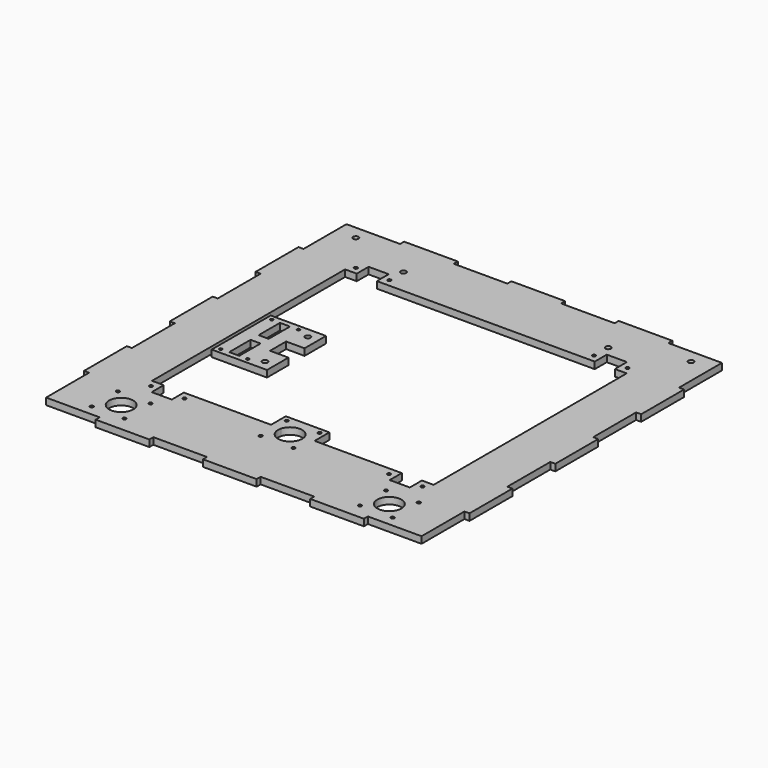
from build123d import *

# Parameters (mm, degrees)
F0_R     = 1.5875
F0_R_2   = 11.43
F0_R_3   = 3.175
F0_W     = 4.7625
F0_H     = 50.8
F0_W_2   = 50.8
F0_H_2   = 4.7625
F0_W_3   = 44.45
F0_H_3   = 41.1268851364
F1_DEPTH = 6.35
F0_R_4   = 1.8415
F0_W_4   = 9.525
F0_H_4   = 25.273
F0_W_5   = 17.4625
F0_H_5   = 25.4
F2_D     = 2.7051
F3_D     = 5.1054
F4_D     = 5.1054


# Not quite as in the source:
# - a feature names something its author has since deleted; it is built from what else it names


with BuildPart() as f1:
    # F0 (on Top) → F1 (new body)
    with BuildSketch(Plane.XY):
        with BuildLine():
            ThreePointArc((155.575, 171.45), (158.75, 174.625), (161.925, 171.45))
            Line((161.925, 171.45), (177.8, 171.45))
            Line((177.8, 171.45), (177.8, 184.15))
            Line((177.8, 184.15), (127, 184.15))
            Line((127, 184.15), (76.2, 184.15))
            Line((76.2, 184.15), (25.4, 184.15))
            Line((25.4, 184.15), (-25.4, 184.15))
            Line((-25.4, 184.15), (-76.2, 184.15))
            Line((-76.2, 184.15), (-127, 184.15))
            Line((-127, 184.15), (-177.8, 184.15))
            Line((-177.8, 184.15), (-177.8, 171.45))
            Line((-177.8, 171.45), (-161.925, 171.45))
            ThreePointArc((-161.925, 171.45), (-158.75, 174.625), (-155.575, 171.45))
            Line((-155.575, 171.45), (155.575, 171.45))
        make_face()
        with BuildLine():
            ThreePointArc((155.575, 171.45), (158.75, 168.275), (161.925, 171.45))
            Line((161.925, 171.45), (155.575, 171.45))
        make_face()
        with BuildLine():
            Line((155.575, 171.45), (161.925, 171.45))
            ThreePointArc((161.925, 171.45), (158.75, 174.625), (155.575, 171.45))
        make_face()
        with BuildLine():
            Line((177.8, 171.45), (161.925, 171.45))
            ThreePointArc((161.925, 171.45), (158.75, 168.275), (155.575, 171.45))
            Line((155.575, 171.45), (-155.575, 171.45))
            ThreePointArc((-155.575, 171.45), (-158.75, 168.275), (-161.925, 171.45))
            Line((-161.925, 171.45), (-177.8, 171.45))
            Line((-177.8, 171.45), (-177.8, 133.35))
            Line((-177.8, 133.35), (-177.8, 82.55))
            Line((-177.8, 82.55), (-177.8, 31.75))
            Line((-177.8, 31.75), (-177.8, -19.05))
            Line((-177.8, -19.05), (-177.8, -69.85))
            Line((-177.8, -69.85), (-177.8, -120.65))
            Line((-177.8, -120.65), (-177.8, -171.45))
            Line((-177.8, -171.45), (-127, -171.45))
            Line((-127, -171.45), (-76.2, -171.45))
            Line((-76.2, -171.45), (-25.4, -171.45))
            Line((-25.4, -171.45), (25.4, -171.45))
            Line((25.4, -171.45), (76.2, -171.45))
            Line((76.2, -171.45), (127, -171.45))
            Line((127, -171.45), (177.8, -171.45))
            Line((177.8, -171.45), (177.8, -120.65))
            Line((177.8, -120.65), (177.8, -69.85))
            Line((177.8, -69.85), (177.8, -19.05))
            Line((177.8, -19.05), (177.8, 31.75))
            Line((177.8, 31.75), (177.8, 82.55))
            Line((177.8, 82.55), (177.8, 133.35))
            Line((177.8, 133.35), (177.8, 171.45))
        make_face()
        with Locations((-142.494, -161.544)):
            Circle(F0_R, mode=Mode.SUBTRACT)
        with Locations((-111.506, -161.544)):
            Circle(F0_R, mode=Mode.SUBTRACT)
        with Locations((-127, -146.05)):
            Circle(F0_R_2, mode=Mode.SUBTRACT)
        with Locations((-142.494, -130.556)):
            Circle(F0_R, mode=Mode.SUBTRACT)
        with Locations((-128.5875, -108.7501)):
            Circle(F0_R, mode=Mode.SUBTRACT)
        with Locations((-111.506, -130.556)):
            Circle(F0_R, mode=Mode.SUBTRACT)
        with Locations((-96.8375, -108.7501)):
            Circle(F0_R, mode=Mode.SUBTRACT)
        with Locations((111.506, -161.544)):
            Circle(F0_R, mode=Mode.SUBTRACT)
        with Locations((127, -146.05)):
            Circle(F0_R_2, mode=Mode.SUBTRACT)
        with Locations((142.494, -161.544)):
            Circle(F0_R, mode=Mode.SUBTRACT)
        with Locations((111.506, -130.556)):
            Circle(F0_R, mode=Mode.SUBTRACT)
        with Locations((96.8375, -108.7501)):
            Circle(F0_R, mode=Mode.SUBTRACT)
        with Locations((128.5875, -108.7501)):
            Circle(F0_R, mode=Mode.SUBTRACT)
        with Locations((142.494, -130.556)):
            Circle(F0_R, mode=Mode.SUBTRACT)
        with Locations((-128.7030479432, 133.9005806915)):
            Circle(F0_R, mode=Mode.SUBTRACT)
        with Locations((-96.9530623423, 133.9308187798)):
            Circle(F0_R, mode=Mode.SUBTRACT)
        with Locations((-96.9530623423, 150.6059263422)):
            Circle(F0_R_3, mode=Mode.SUBTRACT)
        Polygon((-122.2375, -101.6), (-133.35, -101.6), (-133.35, 126.746051779), (-133.35, 127), (-122.3464730803, 127), (-122.3598604405, 141.0567250664), (-103.30986908, 141.0748679195), (-103.2964644408, 127), (-22.225, 127), (-22.225, 168.1268851364), (22.225, 168.1268851364), (22.225, 127), (103.0786291533, 127), (103.065037326, 141.2714154939), (122.1150286865, 141.289558347), (122.1286377928, 127), (133.2411428818, 127), (133.35, 127), (133.35, -101.6), (122.2375, -101.6), (122.2375, -115.9002), (103.1875, -115.9002), (103.1875, -101.6), (20.6375, -101.6), (20.6375, -125.4125), (-20.6375, -125.4125), (-20.6375, -101.6), (-103.1875, -101.6), (-103.1875, -115.9002), (-122.2375, -115.9002), align=None, mode=Mode.SUBTRACT)
        with Locations((96.7218498233, 134.115271119)):
            Circle(F0_R, mode=Mode.SUBTRACT)
        with Locations((128.4718354242, 134.1455092073)):
            Circle(F0_R, mode=Mode.SUBTRACT)
        with Locations((96.9530623423, 150.6059263422)):
            Circle(F0_R_3, mode=Mode.SUBTRACT)
        with Locations((180.18125, 107.95)):
            Rectangle(F0_W, F0_H)
        with BuildLine():
            ThreePointArc((-161.925, 171.45), (-158.75, 168.275), (-155.575, 171.45))
            Line((-155.575, 171.45), (-161.925, 171.45))
        make_face()
        with BuildLine():
            Line((-161.925, 171.45), (-155.575, 171.45))
            ThreePointArc((-155.575, 171.45), (-158.75, 174.625), (-161.925, 171.45))
        make_face()
        with Locations((101.6, 186.53125)):
            Rectangle(F0_W_2, F0_H_2)
        with Locations((180.18125, 6.35)):
            Rectangle(F0_W, F0_H)
        with Locations((0, 186.53125)):
            Rectangle(F0_W_2, F0_H_2)
        with Locations((-180.18125, 107.95)):
            Rectangle(F0_W, F0_H)
        with Locations((180.18125, -95.25)):
            Rectangle(F0_W, F0_H)
        with Locations((-101.6, 186.53125)):
            Rectangle(F0_W_2, F0_H_2)
        with Locations((-180.18125, 6.35)):
            Rectangle(F0_W, F0_H)
        with Locations((101.6, -173.83125)):
            Rectangle(F0_W_2, F0_H_2)
        with Locations((-180.18125, -95.25)):
            Rectangle(F0_W, F0_H)
        with Locations((0, -173.83125)):
            Rectangle(F0_W_2, F0_H_2)
        with Locations((-101.6, -173.83125)):
            Rectangle(F0_W_2, F0_H_2)
        with BuildLine():
            Line((-20.6375, -84.1375), (-20.6375, -101.6))
            Line((-20.6375, -101.6), (-10.9801764558, -101.6))
            ThreePointArc((-10.9801764558, -101.6), (0, -93.345), (10.9801764558, -101.6))
            Line((10.9801764558, -101.6), (20.6375, -101.6))
            Line((20.6375, -101.6), (20.6375, -84.1375))
            Line((20.6375, -84.1375), (-20.6375, -84.1375))
        make_face()
        with Locations((-15.494, -89.281)):
            Circle(F0_R, mode=Mode.SUBTRACT)
        with Locations((15.494, -89.281)):
            Circle(F0_R, mode=Mode.SUBTRACT)
        with BuildLine():
            Line((-10.9801764558, -101.6), (-20.6375, -101.6))
            Line((-20.6375, -101.6), (-20.6375, -125.4125))
            Line((-20.6375, -125.4125), (20.6375, -125.4125))
            Line((20.6375, -125.4125), (20.6375, -101.6))
            Line((20.6375, -101.6), (10.9801764558, -101.6))
            ThreePointArc((10.9801764558, -101.6), (11.3169853956, -103.1716467778), (11.43, -104.775))
            ThreePointArc((11.43, -104.775), (-1.6033532222, -116.0919853956), (-10.9801764558, -101.6))
        make_face()
        with Locations((-15.494, -120.269)):
            Circle(F0_R, mode=Mode.SUBTRACT)
        with Locations((15.494, -120.269)):
            Circle(F0_R, mode=Mode.SUBTRACT)
        with Locations((0, 147.5634425682)):
            Rectangle(F0_W_3, F0_H_3)
        with Locations((-96.9530623423, 150.6059263422)):
            Circle(F0_R_3)
        with Locations((96.9530623423, 150.6059263422)):
            Circle(F0_R_3)
    extrude(amount=F1_DEPTH)

    # F4 (through all)
    with Locations(Plane(origin=(0, 0, 0), x_dir=(1, 0, 0), z_dir=(0, 0, -1))):
        with Locations((-158.75, -171.45), (-96.9530623423, -150.6059263422), (96.9530623423, -150.6059263422), (158.75, -171.45)):
            Hole(F4_D / 2)


with BuildPart() as f1b:
    # F0 (on Top) → F1, piece 2 (new body)
    with BuildSketch(Plane.XY):
        Polygon((-100.0125, 34.925), (-130.175, 34.925), (-130.175, -34.925), (-100.0125, -34.925), (-95.25, -34.925), (-95.25, -9.525), (-95.25, 9.525), (-95.25, 34.925), align=None)
        with Locations((-125.4125, -30.1625)):
            Circle(F0_R_4, mode=Mode.SUBTRACT)
        with Locations((-100.0125, -30.1625)):
            Circle(F0_R_4, mode=Mode.SUBTRACT)
        with Locations((-112.7125, -17.399)):
            Rectangle(F0_W_4, F0_H_4, mode=Mode.SUBTRACT)
        with Locations((-112.7125, 17.399)):
            Rectangle(F0_W_4, F0_H_4, mode=Mode.SUBTRACT)
        with Locations((-125.4125, 30.1625)):
            Circle(F0_R_4, mode=Mode.SUBTRACT)
        with Locations((-100.0125, 30.1625)):
            Circle(F0_R_4, mode=Mode.SUBTRACT)
        with Locations((-86.51875, 22.225)):
            Rectangle(F0_W_5, F0_H_5)
        with Locations((-87.3125, 25.4)):
            Circle(F0_R_3, mode=Mode.SUBTRACT)
        with Locations((-86.51875, -22.225)):
            Rectangle(F0_W_5, F0_H_5)
        with Locations((-87.3125, -25.4)):
            Circle(F0_R_3, mode=Mode.SUBTRACT)
        with Locations((-87.3125, 25.4)):
            Circle(F0_R_3)
        with Locations((-87.3125, -25.4)):
            Circle(F0_R_3)
        with Locations((-125.4125, 30.1625)):
            Circle(F0_R_4)
        with Locations((-100.0125, 30.1625)):
            Circle(F0_R_4)
        with Locations((-125.4125, -30.1625)):
            Circle(F0_R_4)
        with Locations((-100.0125, -30.1625)):
            Circle(F0_R_4)
    extrude(amount=F1_DEPTH)

    # F2 (through all)
    with Locations(Plane(origin=(0, 0, 0), x_dir=(1, 0, 0), z_dir=(0, 0, -1))):
        with Locations((-125.4125, -30.1625), (-100.0125, -30.1625), (-100.0125, 30.1625), (-125.4125, 30.1625)):
            Hole(F2_D / 2)

    # F3 (through all)
    with Locations(Plane(origin=(0, 0, 0), x_dir=(1, 0, 0), z_dir=(0, 0, -1))):
        with Locations((-87.3125, -25.4), (-87.3125, 25.4)):
            Hole(F3_D / 2)


solid = Compound([f1.part, f1b.part])
